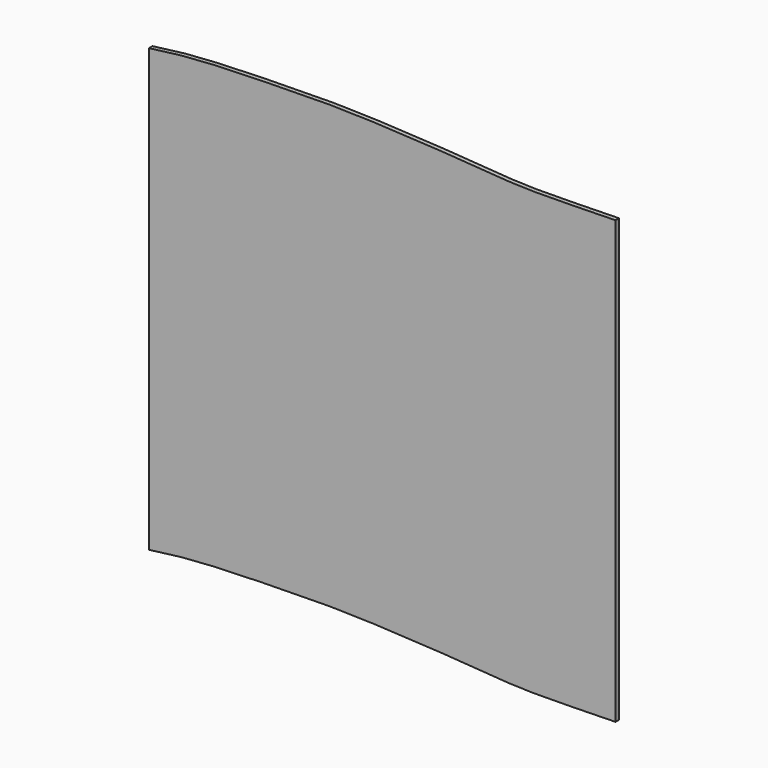
from build123d import *

# Parameters (mm, degrees)
F1_DEPTH = 3


# Not quite as in the source:
# - the dataset's text gives a spline's control points without its knots; the knots are read off the source's solid


with BuildPart() as f1:
    # F0 (on Front) → F1 (new body)
    with BuildSketch(Plane.XZ):
        with BuildLine():
            add(Edge.make_bspline(
                [(0, 0), (2.2836279369, 0.3145032409), (6.8468695701, 0.9430212827), (13.7883957694, 1.843023423), (20.9351718591, 2.6617660327), (28.4000924164, 3.352293114), (36.2889316073, 3.9112052115), (43.2725801473, 4.2918421707), (49.1423870677, 4.5562734212), (53.6953625842, 4.7376825434), (58.4071616109, 4.9050635606), (63.2902761656, 5.0616060673), (68.3075293089, 5.2076702034), (75.1176202129, 5.3884210069), (82.024215434, 5.5483277484), (88.8576319072, 5.6876320865), (93.9038556027, 5.7818708045), (98.8285547302, 5.8659479641), (103.5906057144, 5.9398743656), (108.1430811393, 6.0039156213), (112.4612934577, 6.0573519358), (116.6453916848, 6.0948291734), (122.1619616105, 6.1171117414), (127.7674711212, 6.0879897124), (133.8243459683, 5.987730754), (138.6831596477, 5.8720051249), (143.0713489502, 5.7376203302), (146.8295178196, 5.604915141), (150.7710511797, 5.4543814812), (156.0371681528, 5.2332504261), (162.7851432075, 4.9226726022), (169.8564474069, 4.5738817065), (179.5727208922, 4.0674021471), (191.9909197151, 3.3743996448), (204.0607844537, 2.6489586812), (213.0804507845, 2.0776092898), (219.4202128983, 1.660722706), (224.2600201136, 1.3289486164), (227.812323813, 1.0764850666), (230.3031695378, 0.8945155465), (232.6078059914, 0.7208213242), (234.7101690311, 0.5563368187), (236.6343126707, 0.4011209176), (239.0002413484, 0.2066110814), (241.6520027599, -0.0130478298), (244.565343726, -0.2384073924), (247.4264911207, -0.424302615), (250.4456840711, -0.5692062647), (253.8395863669, -0.6718571), (257.8014120165, -0.7317828333), (262.2687110809, -0.7533390738), (267.1958040678, -0.7403987813), (272.5313211273, -0.6968519806), (280.122623956, -0.6031018214), (290.3791232139, -0.4285877374), (303.5055932591, -0.1580584898), (312.528848624, 0.0426461204), (317.0400871915, 0.1429895898)],
                knots=[0, 0, 0, 0, 0.03125, 0.0625, 0.09375, 0.125, 0.15625, 0.1875, 0.203125, 0.21875, 0.234375, 0.25, 0.265625, 0.28125, 0.3125, 0.328125, 0.34375, 0.359375, 0.375, 0.390625, 0.40625, 0.421875, 0.4375, 0.46875, 0.484375, 0.5, 0.515625, 0.5234375, 0.53125, 0.546875, 0.5625, 0.578125, 0.59375, 0.625, 0.65625, 0.671875, 0.6875, 0.703125, 0.7109375, 0.71875, 0.7265625, 0.734375, 0.7421875, 0.75, 0.765625, 0.78125, 0.796875, 0.8125, 0.828125, 0.84375, 0.859375, 0.875, 0.890625, 0.90625, 0.9375, 0.96875, 1, 1, 1, 1], degree=3))
            Line((0, 0), (0, -300))
            add(Edge.make_bspline(
                [(0, -300), (2.2836279369, -299.6854967591), (6.8468695701, -299.0569787173), (13.7883957694, -298.156976577), (20.9351718591, -297.3382339673), (28.4000924164, -296.647706886), (36.2889316073, -296.0887947885), (43.2725801473, -295.7081578293), (49.1423870677, -295.4437265788), (53.6953625842, -295.2623174566), (58.4071616109, -295.0949364394), (63.2902761656, -294.9383939327), (68.3075293089, -294.7923297966), (75.1176202129, -294.6115789931), (82.024215434, -294.4516722516), (88.8576319072, -294.3123679135), (93.9038556027, -294.2181291955), (98.8285547302, -294.1340520359), (103.5906057144, -294.0601256344), (108.1430811393, -293.9960843787), (112.4612934577, -293.9426480642), (116.6453916848, -293.9051708266), (122.1619616105, -293.8828882586), (127.7674711212, -293.9120102876), (133.8243459683, -294.012269246), (138.6831596477, -294.1279948751), (143.0713489502, -294.2623796698), (146.8295178196, -294.395084859), (150.7710511797, -294.5456185188), (156.0371681528, -294.7667495739), (162.7851432075, -295.0773273978), (169.8564474069, -295.4261182935), (179.5727208922, -295.9325978529), (191.9909197151, -296.6256003552), (204.0607844537, -297.3510413188), (213.0804507845, -297.9223907102), (219.4202128983, -298.339277294), (224.2600201136, -298.6710513836), (227.812323813, -298.9235149334), (230.3031695378, -299.1054844535), (232.6078059914, -299.2791786758), (234.7101690311, -299.4436631813), (236.6343126707, -299.5988790824), (239.0002413484, -299.7933889186), (241.6520027599, -300.0130478298), (244.565343726, -300.2384073924), (247.4264911207, -300.424302615), (250.4456840711, -300.5692062647), (253.8395863669, -300.6718571), (257.8014120165, -300.7317828333), (262.2687110809, -300.7533390738), (267.1958040678, -300.7403987813), (272.5313211273, -300.6968519806), (280.122623956, -300.6031018214), (290.3791232139, -300.4285877374), (303.5055932591, -300.1580584898), (312.528848624, -299.9573538796), (317.0400871915, -299.8570104102)],
                knots=[0, 0, 0, 0, 0.03125, 0.0625, 0.09375, 0.125, 0.15625, 0.1875, 0.203125, 0.21875, 0.234375, 0.25, 0.265625, 0.28125, 0.3125, 0.328125, 0.34375, 0.359375, 0.375, 0.390625, 0.40625, 0.421875, 0.4375, 0.46875, 0.484375, 0.5, 0.515625, 0.5234375, 0.53125, 0.546875, 0.5625, 0.578125, 0.59375, 0.625, 0.65625, 0.671875, 0.6875, 0.703125, 0.7109375, 0.71875, 0.7265625, 0.734375, 0.7421875, 0.75, 0.765625, 0.78125, 0.796875, 0.8125, 0.828125, 0.84375, 0.859375, 0.875, 0.890625, 0.90625, 0.9375, 0.96875, 1, 1, 1, 1], degree=3))
            Line((317.0400871915, -299.8570104102), (317.0400871915, 0.1429895898))
        make_face()
    extrude(amount=F1_DEPTH)


solid = f1.part
